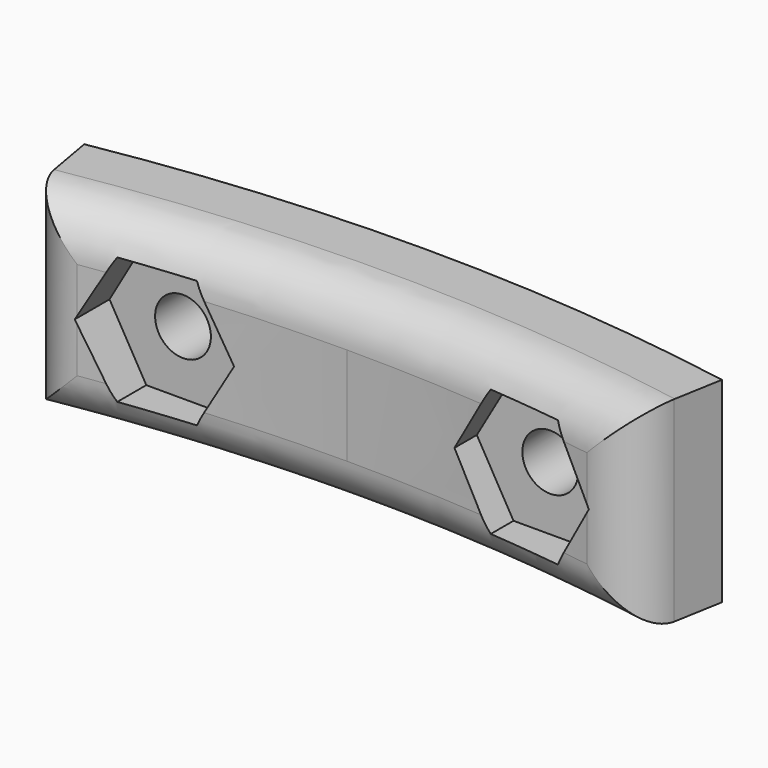
from build123d import *

# Parameters (mm, degrees)
F1_DEPTH     = 10.16
F5_R         = 1.4478
F6_DEPTH     = 25.4
F10_DEPTH    = 1.27
F11_T1_DEPTH = 22.6859947386
F11_T4_ANGLE = 28.0699881424
F11_T6_ANGLE = 28.0699881424


# Not quite as in the source:
# - a fillet or chamfer that OpenCascade refuses, or shapes differently, is made with other operations: its cross-section is extruded or revolved along the edge and cut away or added


with BuildPart() as f1:
    # F0 (on Top) → F1 (new body)
    with BuildSketch(Plane.XY):
        with BuildLine():
            ThreePointArc((0, 95.25), (-8.3015844967, 94.8875449932), (-16.5399889228, 93.8029384744))
            Line((-16.5399889228, 93.8029384744), (-15.6578561802, 88.8001150891))
            ThreePointArc((-15.6578561802, 88.8001150891), (-7.8588333236, 89.8268759269), (0, 90.17))
            Line((0, 90.17), (0, 95.25))
        make_face()
        with BuildLine():
            Line((15.6578561802, 88.8001150891), (16.5399889228, 93.8029384744))
            ThreePointArc((16.5399889228, 93.8029384744), (8.3015844967, 94.8875449932), (0, 95.25))
            Line((0, 95.25), (0, 90.17))
            ThreePointArc((0, 90.17), (7.8588333236, 89.8268759269), (15.6578561802, 88.8001150891))
        make_face()
    extrude(amount=F1_DEPTH)

    # F5 (on line) → F6 (cut)
    with BuildSketch(Plane(origin=(0, 95.25, 0), x_dir=(-1, 0, 0), z_dir=(0, 1, 0))):
        with Locations((-9.525, 5.08)):
            Circle(F5_R)
        with BuildLine():
            ThreePointArc((10.9728, 5.08), (9.525, 6.5278), (8.0772, 5.08))
            ThreePointArc((8.0772, 5.08), (9.525, 3.6322), (10.9728, 5.08))
        make_face()
    extrude(amount=-F6_DEPTH, mode=Mode.SUBTRACT)

    # F9 (on line) → F10 (cut, symmetric)
    with BuildSketch(Plane(origin=(0, 90.17, 0), x_dir=(-1, 0, 0), z_dir=(0, 1, 0))):
        Polygon((7.62, 8.3795567884), (5.715, 5.08), (7.62, 1.7804432116), (11.43, 1.7804432116), (13.335, 5.08), (11.43, 8.3795567884), align=None)
        Polygon((-11.43, 8.3795567884), (-13.335, 5.08), (-11.43, 1.7804432116), (-7.62, 1.7804432116), (-5.715, 5.08), (-7.62, 8.3795567884), align=None)
    extrude(amount=F10_DEPTH, both=True, mode=Mode.SUBTRACT)

    # F11: fillet of radius 2.54 on 4 edges, made by hand

    # F11_s2 → F11_t1 (cut)
    with BuildSketch(Plane.XY.offset(-6.2629973693)):
        with BuildLine():
            ThreePointArc((13.2190987409, 89.1957640725), (15.0767198196, 89.6478290697), (16.0928794122, 91.2672544357))
            Line((16.0928794122, 91.2672544357), (15.6578561802, 88.8001150891))
            ThreePointArc((15.6578561802, 88.8001150891), (14.4398326136, 89.0062926657), (13.2190987409, 89.1957640725))
        make_face()
        with BuildLine():
            ThreePointArc((-16.0928794122, 91.2672544357), (-15.0767198196, 89.6478290697), (-13.2190987409, 89.1957640725))
            ThreePointArc((-13.2190987409, 89.1957640725), (-14.4398326136, 89.0062926657), (-15.6578561802, 88.8001150891))
            Line((-15.6578561802, 88.8001150891), (-16.0928794122, 91.2672544357))
        make_face()
    extrude(amount=F11_T1_DEPTH, mode=Mode.SUBTRACT)

    # F11_s3 → F11_t4 (revolve, cut)
    with BuildSketch(Plane(origin=(0, 0, 0), x_dir=(0, 0, 1), z_dir=(-0.9701477887, -0.24251447, 0))):
        with BuildLine():
            ThreePointArc((7.62, 90.17), (9.4160512242, 90.9139487758), (10.16, 92.71))
            Line((10.16, 92.71), (10.16, 90.17))
            Line((10.16, 90.17), (7.62, 90.17))
        make_face()
    revolve(axis=Axis((0, 0, 10.16), (0, 0, -1)), revolution_arc=F11_T4_ANGLE, mode=Mode.SUBTRACT)

    # F11_s5 → F11_t6 (revolve, cut)
    with BuildSketch(Plane(origin=(0, 0, 0), x_dir=(0, 0, 1), z_dir=(-0.9701477887, -0.24251447, 0))):
        with BuildLine():
            ThreePointArc((2.54, 90.17), (0.7439487758, 90.9139487758), (0, 92.71))
            Line((0, 92.71), (0, 90.17))
            Line((0, 90.17), (2.54, 90.17))
        make_face()
    revolve(axis=Axis((0, 0, 0), (0, 0, -1)), revolution_arc=F11_T6_ANGLE, mode=Mode.SUBTRACT)


solid = f1.part
